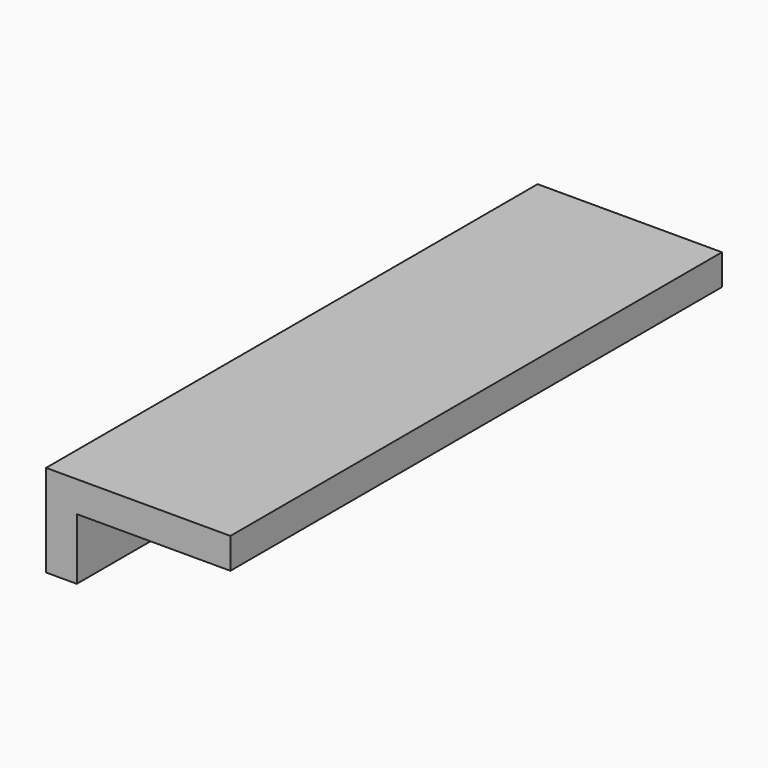
from build123d import *

# Parameters (mm, degrees)
F1_DEPTH = 50
F3_D     = 3.5
F4_R     = 2.4
F4_R_2   = 1.75
F5_DEPTH = 2


with BuildPart() as f1:
    # F0 (on Front) → F1 (new body, symmetric)
    with BuildSketch(Plane.XZ):
        Polygon((-9.9684563031, 8.1134089709), (-9.9684563031, -6.8865910291), (-4.9684563031, -6.8865910291), (-4.9684563031, 3.1134089709), (20.0315436969, 3.1134089709), (20.0315436969, 8.1134089709), align=None)
    extrude(amount=F1_DEPTH, both=True)

    # F3 (through all)
    with Locations(Plane.YZ.offset(-4.9684563031)):
        with Locations((-25, -1.8865910291), (25, -1.8865910291)):
            Hole(F3_D / 2)

    # F4 (on face) → F5 (cut)
    with BuildSketch(Plane.YZ.offset(-4.9684563031)):
        with Locations((-25, -1.8865910291)):
            Circle(F4_R)
        with Locations((-25, -1.8865910291)):
            Circle(F4_R_2, mode=Mode.SUBTRACT)
        with Locations((25, -1.8865910291)):
            Circle(F4_R)
        with Locations((25, -1.8865910291)):
            Circle(F4_R_2, mode=Mode.SUBTRACT)
    extrude(amount=-F5_DEPTH, mode=Mode.SUBTRACT)


solid = f1.part
